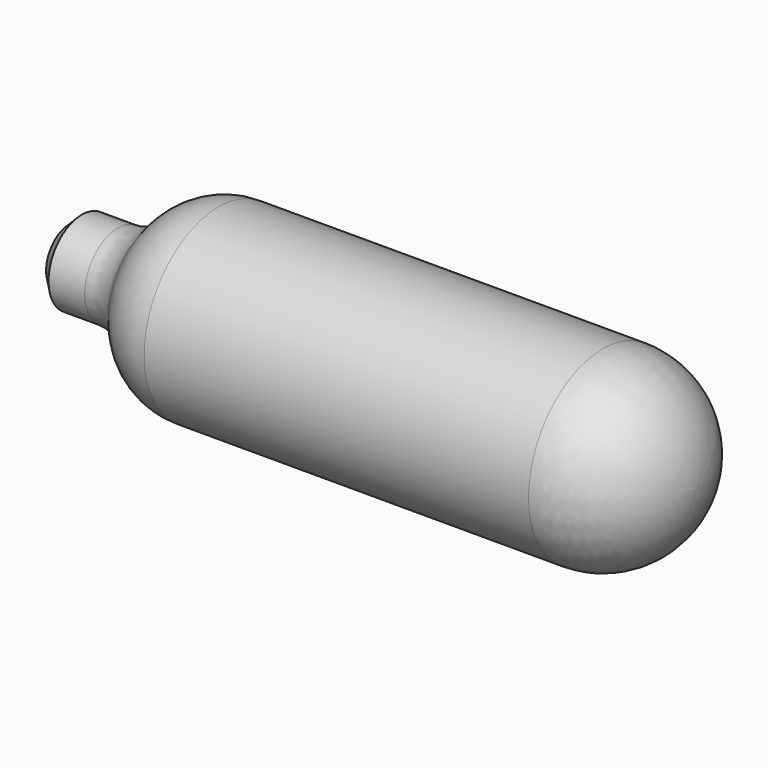
from build123d import *

# Parameters (mm, degrees)
F3_R    = 5.08
F4_SIZE = 1.27


# Not quite as in the source:
# - a fillet or chamfer that OpenCascade refuses, or shapes differently, is made with other operations: its cross-section is extruded or revolved along the edge and cut away or added


with BuildPart() as f1:
    # F0 (on Front) → F1 (revolve)
    with BuildSketch(Plane.XZ):
        with BuildLine():
            Line((-65.912999015, 22.4110006839), (-65.912999015, 18.1610006839))
            Line((-65.912999015, 18.1610006839), (-1.912999015, 18.1610006839))
            Line((-1.912999015, 18.1610006839), (-1.912999015, 18.1654242131))
            ThreePointArc((-1.912999015, 18.1654242131), (-4.6948756483, 24.8821639675), (-11.4112079773, 27.6650241112))
            Line((-11.4112079773, 27.6650241112), (-57.911999015, 27.6650241112))
            Line((-57.911999015, 27.6650241112), (-57.911999015, 22.4110006839))
            Line((-57.911999015, 22.4110006839), (-65.912999015, 22.4110006839))
        make_face()
    revolve(axis=Axis((-33.912999015, 0, 18.1610006839), (1, 0, 0)))

    # F2: fillet of radius 7.62 on 1 edges, made by hand

    # F2_s1 → F2_t2 (revolve, cut)
    with BuildSketch(Plane.XZ):
        with BuildLine():
            ThreePointArc((-50.6686189437, 27.6650241112), (-55.1427478263, 26.2132143435), (-57.911999015, 22.4110006839))
            Line((-57.911999015, 22.4110006839), (-57.911999015, 27.6650241112))
            Line((-57.911999015, 27.6650241112), (-50.6686189437, 27.6650241112))
        make_face()
    revolve(axis=Axis((-57.911999015, 0, 18.1610006839), (1, 0, 0)), mode=Mode.SUBTRACT)

    # F3
    f3_edges = [f1.edges().sort_by_distance(p)[0] for p in [
        (-57.911999, 0, 13.911001),
    ]]
    fillet(f3_edges, radius=F3_R)

    # F4
    f4_edges = [f1.edges().sort_by_distance(p)[0] for p in [
        (-65.912999, 0, 13.911001),
    ]]
    chamfer(f4_edges, length=F4_SIZE)


solid = f1.part
